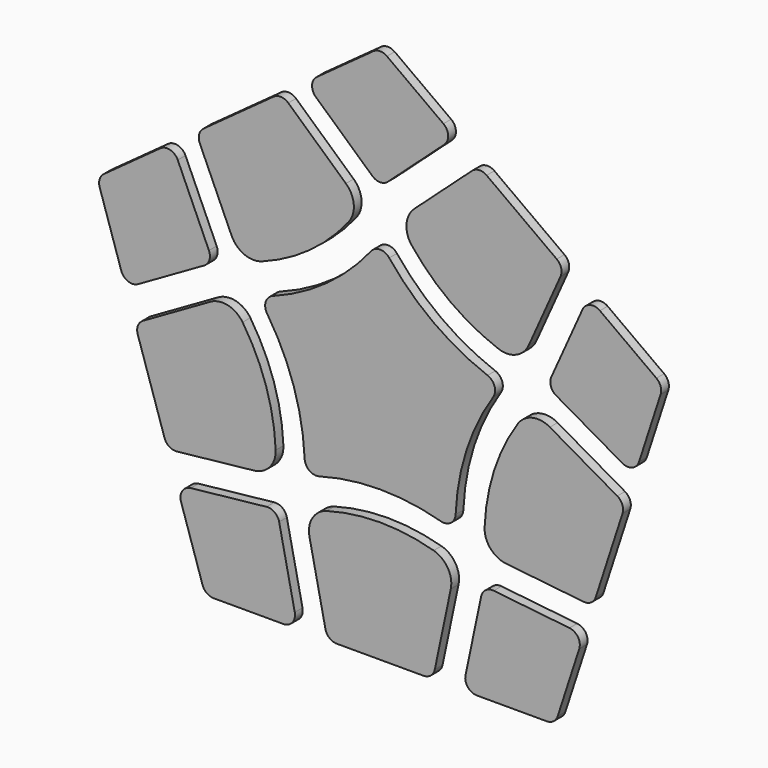
from build123d import *

# Parameters (mm, degrees)
F1_DEPTH = 1


# Not quite as in the source:
# - a feature names something its author has since deleted; it is built from what else it names


with BuildPart() as f1:
    # F0 (on Front) → F1 (new body)
    with BuildSketch(Plane.XZ):
        with BuildLine():
            Line((-17.694116513, 6.5958520163), (-20.9137744033, 13.7776049975))
            ThreePointArc((-20.9137744033, 13.7776049975), (-21.6996777578, 14.4462150283), (-22.7141135884, 14.2575263913))
            Line((-22.7141135884, 14.2575263913), (-28.5494375554, 10.0179153646))
            ThreePointArc((-28.5494375554, 10.0179153646), (-28.9853630722, 9.4179153646), (-28.9853630722, 8.6762745781))
            Line((-28.9853630722, 8.6762745781), (-26.7564676522, 1.8164398378))
            ThreePointArc((-26.7564676522, 1.8164398378), (-26.0466802236, 1.0675171033), (-25.0178719382, 1.1464915793))
            Line((-25.0178719382, 1.1464915793), (-18.191785501, 5.0641843652))
            ThreePointArc((-18.191785501, 5.0641843652), (-17.6478455759, 5.7341326237), (-17.694116513, 6.5958520163))
        make_face()
    extrude(amount=F1_DEPTH)


with BuildPart() as f1b:
    # F0 (on Front) → F1, piece 2 (new body)
    with BuildSketch(Plane.XZ):
        with BuildLine():
            ThreePointArc((-12.2053541777, 7.3856519674), (-7.2800742754, 10.0201626124), (-3.2525105674, 13.8902735969))
            ThreePointArc((-3.2525105674, 13.8902735969), (-2.7235874919, 15.6476925752), (-3.5372825515, 17.2927401232))
            Line((-3.5372825515, 17.2927401232), (-9.4939464638, 22.6839212654))
            ThreePointArc((-9.4939464638, 22.6839212654), (-10.2348492198, 22.9924872502), (-11.0045341042, 22.7650338717))
            Line((-11.0045341042, 22.7650338717), (-18.2502457539, 17.5007162125))
            ThreePointArc((-18.2502457539, 17.5007162125), (-18.7044124814, 16.838989347), (-18.6399003336, 16.0389968198))
            Line((-18.6399003336, 16.0389968198), (-15.3532927565, 8.7079061979))
            ThreePointArc((-15.3532927565, 8.7079061979), (-14.040205168, 7.4256885604), (-12.2053541777, 7.3856519674))
        make_face()
    extrude(amount=F1_DEPTH)


with BuildPart() as f1c:
    # F0 (on Front) → F1, piece 3 (new body)
    with BuildSketch(Plane.XZ):
        with BuildLine():
            Line((0.8052453376, 18.8663351752), (6.6405693046, 24.1476955125))
            ThreePointArc((6.6405693046, 24.1476955125), (7.0335977388, 25.1017458812), (6.5406662698, 26.0082236928))
            Line((6.5406662698, 26.0082236928), (0.7053423028, 30.2478347195))
            ThreePointArc((0.7053423028, 30.2478347195), (0, 30.4770143263), (-0.7053423028, 30.2478347195))
            Line((-0.7053423028, 30.2478347195), (-6.5406662698, 26.0082236928))
            ThreePointArc((-6.5406662698, 26.0082236928), (-7.0335977388, 25.1017458812), (-6.6405693046, 24.1476955125))
            Line((-6.6405693046, 24.1476955125), (-0.8052453376, 18.8663351752))
            ThreePointArc((-0.8052453376, 18.8663351752), (0, 18.5560429622), (0.8052453376, 18.8663351752))
        make_face()
    extrude(amount=F1_DEPTH)


with BuildPart() as f1d:
    # F0 (on Front) → F1, piece 4 (new body)
    with BuildSketch(Plane.XZ):
        with BuildLine():
            ThreePointArc((3.2525105674, 13.8902735969), (7.2800742754, 10.0201626124), (12.2053541777, 7.3856519674))
            ThreePointArc((12.2053541777, 7.3856519674), (14.040205168, 7.4256885604), (15.3532927565, 8.7079061979))
            Line((15.3532927565, 8.7079061979), (18.6399003336, 16.0389968198))
            ThreePointArc((18.6399003336, 16.0389968198), (18.7044124814, 16.838989347), (18.2502457539, 17.5007162125))
            Line((18.2502457539, 17.5007162125), (11.0045341042, 22.7650338717))
            ThreePointArc((11.0045341042, 22.7650338717), (10.2348492198, 22.9924872502), (9.4939464638, 22.6839212654))
            Line((9.4939464638, 22.6839212654), (3.5372825515, 17.2927401232))
            ThreePointArc((3.5372825515, 17.2927401232), (2.7235874919, 15.6476925752), (3.2525105674, 13.8902735969))
        make_face()
    extrude(amount=F1_DEPTH)


with BuildPart() as f1e:
    # F0 (on Front) → F1, piece 5 (new body)
    with BuildSketch(Plane.XZ):
        with BuildLine():
            ThreePointArc((-10.795834294, -9.3256896519), (-11.7794076183, -3.8273615451), (-14.2155162571, 1.1990092285))
            ThreePointArc((-14.2155162571, 1.1990092285), (-15.7234748093, 2.2451172966), (-17.5394536011, 1.9795949568))
            Line((-17.5394536011, 1.9795949568), (-24.5074819356, -2.0195624797))
            ThreePointArc((-24.5074819356, -2.0195624797), (-25.0298971689, -2.6288507405), (-25.0514218607, -3.4311515247))
            Line((-25.0514218607, -3.4311515247), (-22.2838062832, -11.9489964249))
            ThreePointArc((-22.2838062832, -11.9489964249), (-21.7948118729, -12.5854194976), (-21.0140384169, -12.7712760853))
            Line((-21.0140384169, -12.7712760853), (-13.0261393142, -11.9109581221))
            ThreePointArc((-13.0261393142, -11.9109581221), (-11.4009114947, -11.058364655), (-10.795834294, -9.3256896519))
        make_face()
    extrude(amount=F1_DEPTH)


with BuildPart() as f1f:
    # F0 (on Front) → F1, piece 6 (new body)
    with BuildSketch(Plane.XZ):
        with BuildLine():
            Line((-11.7408107436, -14.7898744444), (-19.5659927189, -15.6326673405))
            ThreePointArc((-19.5659927189, -15.6326673405), (-20.4447361381, -16.173493985), (-20.5787604917, -17.1965877874))
            Line((-20.5787604917, -17.1965877874), (-18.3498650717, -24.0564225277))
            ThreePointArc((-18.3498650717, -24.0564225277), (-17.9139395549, -24.6564225277), (-17.2085972521, -24.8856021345))
            Line((-17.2085972521, -24.8856021345), (-9.9957401582, -24.8856021345))
            ThreePointArc((-9.9957401582, -24.8856021345), (-9.0641359335, -24.4419840278), (-8.8213258793, -23.4391247487))
            Line((-8.8213258793, -23.4391247487), (-10.437896418, -15.7364971123))
            ThreePointArc((-10.437896418, -15.7364971123), (-10.9069683941, -15.0121541048), (-11.7408107436, -14.7898744444))
        make_face()
    extrude(amount=F1_DEPTH)


with BuildPart() as f1g:
    # F0 (on Front) → F1, piece 7 (new body)
    with BuildSketch(Plane.XZ):
        with BuildLine():
            ThreePointArc((-5.5331616471, -13.1492451408), (-6.9940543615, -14.2601337772), (-7.3026959181, -16.069283156))
            Line((-7.3026959181, -16.069283156), (-5.652510351, -23.9320795203))
            ThreePointArc((-5.652510351, -23.9320795203), (-5.2344779655, -24.6172063592), (-4.4780960722, -24.8856021345))
            Line((-4.4780960722, -24.8856021345), (4.4780960722, -24.8856021345))
            ThreePointArc((4.4780960722, -24.8856021345), (5.2344779655, -24.6172063592), (5.652510351, -23.9320795203))
            Line((5.652510351, -23.9320795203), (7.3026959181, -16.069283156))
            ThreePointArc((7.3026959181, -16.069283156), (6.9940543615, -14.2601337772), (5.5331616471, -13.1492451408))
            ThreePointArc((5.5331616471, -13.1492451408), (0, -12.3856021345), (-5.5331616471, -13.1492451408))
        make_face()
    extrude(amount=F1_DEPTH)


with BuildPart() as f1h:
    # F0 (on Front) → F1, piece 8 (new body)
    with BuildSketch(Plane.XZ):
        with BuildLine():
            Line((10.437896418, -15.7364971123), (8.8213258793, -23.4391247487))
            ThreePointArc((8.8213258793, -23.4391247487), (9.0641359335, -24.4419840278), (9.9957401582, -24.8856021345))
            Line((9.9957401582, -24.8856021345), (17.2085972521, -24.8856021345))
            ThreePointArc((17.2085972521, -24.8856021345), (17.9139395549, -24.6564225277), (18.3498650717, -24.0564225277))
            Line((18.3498650717, -24.0564225277), (20.5787604917, -17.1965877874))
            ThreePointArc((20.5787604917, -17.1965877874), (20.4447361381, -16.173493985), (19.5659927189, -15.6326673405))
            Line((19.5659927189, -15.6326673405), (11.7408107436, -14.7898744444))
            ThreePointArc((11.7408107436, -14.7898744444), (10.9069683941, -15.0121541048), (10.437896418, -15.7364971123))
        make_face()
    extrude(amount=F1_DEPTH)


with BuildPart() as f1i:
    # F0 (on Front) → F1, piece 9 (new body)
    with BuildSketch(Plane.XZ):
        with BuildLine():
            ThreePointArc((14.2155162571, 1.1990092285), (11.7794076183, -3.8273615451), (10.795834294, -9.3256896519))
            ThreePointArc((10.795834294, -9.3256896519), (11.4009114947, -11.058364655), (13.0261393142, -11.9109581221))
            Line((13.0261393142, -11.9109581221), (21.0140384169, -12.7712760853))
            ThreePointArc((21.0140384169, -12.7712760853), (21.7948118729, -12.5854194976), (22.2838062832, -11.9489964249))
            Line((22.2838062832, -11.9489964249), (25.0514218607, -3.4311515247))
            ThreePointArc((25.0514218607, -3.4311515247), (25.0298971689, -2.6288507405), (24.5074819356, -2.0195624797))
            Line((24.5074819356, -2.0195624797), (17.5394536011, 1.9795949568))
            ThreePointArc((17.5394536011, 1.9795949568), (15.7234748093, 2.2451172966), (14.2155162571, 1.1990092285))
        make_face()
    extrude(amount=F1_DEPTH)


with BuildPart() as f1j:
    # F0 (on Front) → F1, piece 10 (new body)
    with BuildSketch(Plane.XZ):
        with BuildLine():
            Line((18.191785501, 5.0641843652), (25.0178719382, 1.1464915793))
            ThreePointArc((25.0178719382, 1.1464915793), (26.0466802236, 1.0675171033), (26.7564676522, 1.8164398378))
            Line((26.7564676522, 1.8164398378), (28.9853630722, 8.6762745781))
            ThreePointArc((28.9853630722, 8.6762745781), (28.9853630722, 9.4179153646), (28.5494375554, 10.0179153646))
            Line((28.5494375554, 10.0179153646), (22.7141135884, 14.2575263913))
            ThreePointArc((22.7141135884, 14.2575263913), (21.6996777578, 14.4462150283), (20.9137744033, 13.7776049975))
            Line((20.9137744033, 13.7776049975), (17.694116513, 6.5958520163))
            ThreePointArc((17.694116513, 6.5958520163), (17.6478455759, 5.7341326237), (18.191785501, 5.0641843652))
        make_face()
    extrude(amount=F1_DEPTH)


with BuildPart() as f1k:
    # F0 (on Front) → F1, piece 11 (new body)
    with BuildSketch(Plane.XZ):
        with BuildLine():
            ThreePointArc((-6.2804257648, -10.2431120979), (0, -9.3856021345), (6.2804257648, -10.2431120979))
            ThreePointArc((6.2804257648, -10.2431120979), (7.3074595861, -10.0578552589), (7.8010202146, -9.1383355623))
            ThreePointArc((7.8010202146, -9.1383355623), (8.9262380694, -2.900310562), (11.6825368011, 2.8077441352))
            ThreePointArc((11.6825368011, 2.8077441352), (11.8237179817, 3.841758855), (11.1017214044, 4.5953101198))
            ThreePointArc((11.1017214044, 4.5953101198), (5.5167185185, 7.5931116293), (0.939779053, 11.9783934052))
            ThreePointArc((0.939779053, 11.9783934052), (0, 12.4321928078), (-0.939779053, 11.9783934052))
            ThreePointArc((-0.939779053, 11.9783934052), (-5.5167185185, 7.5931116293), (-11.1017214044, 4.5953101198))
            ThreePointArc((-11.1017214044, 4.5953101198), (-11.8237179817, 3.841758855), (-11.6825368011, 2.8077441352))
            ThreePointArc((-11.6825368011, 2.8077441352), (-8.9262380694, -2.900310562), (-7.8010202146, -9.1383355623))
            ThreePointArc((-7.8010202146, -9.1383355623), (-7.3074595861, -10.0578552589), (-6.2804257648, -10.2431120979))
        make_face()
    extrude(amount=F1_DEPTH)


solid = Compound([f1.part, f1b.part, f1c.part, f1d.part, f1e.part, f1f.part, f1g.part, f1h.part, f1i.part, f1j.part, f1k.part])
